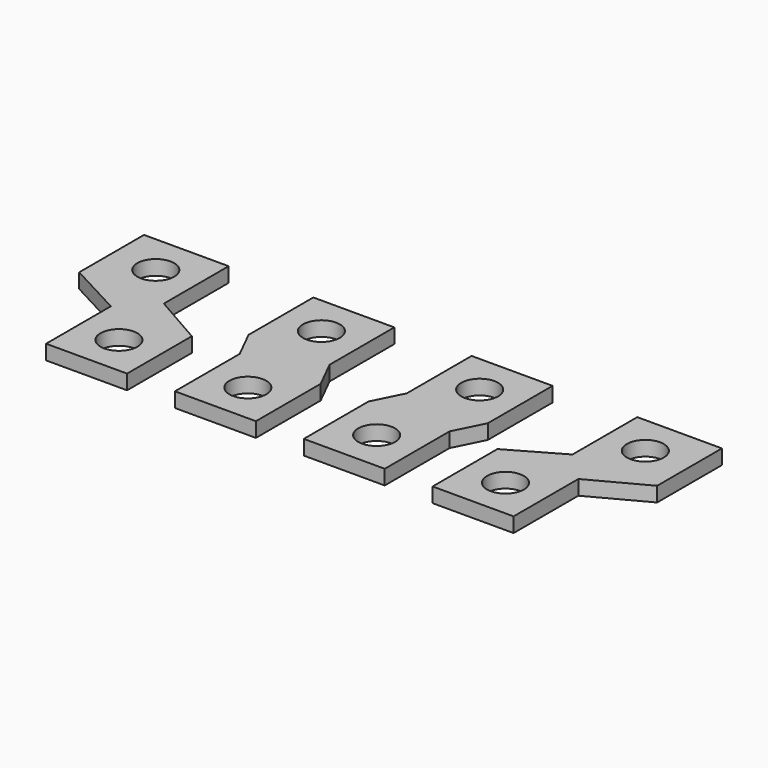
from build123d import *

# Parameters (mm, degrees)
F0_R     = 5
F1_DEPTH = 4


# Not quite as in the source:
# - a feature names something its author has since deleted; it is built from what else it names


with BuildPart() as f1:
    # F0 (on Top) → F1 (new body)
    with BuildSketch(Plane.XY):
        Polygon((-33.4400572926, 67.2019907534), (-56.4400572926, 67.2019907534), (-56.4400572926, 45.2019907534), (-41.4400572926, 37.2019907534), (-41.4400572926, 15.2019907534), (-19.4400572926, 15.2019907534), (-19.4400572926, 37.2019907534), (-33.4400572926, 45.2019907534), align=None)
        with Locations((-30.4400572926, 26.2019907534)):
            Circle(F0_R, mode=Mode.SUBTRACT)
        with Locations((-44.4400572926, 56.2019907534)):
            Circle(F0_R, mode=Mode.SUBTRACT)
    extrude(amount=F1_DEPTH)


with BuildPart() as f1b:
    # F0 (on Top) → F1, piece 2 (new body)
    with BuildSketch(Plane.XY):
        Polygon((11.5599427074, 67.2019907534), (-10.4400572926, 67.2019907534), (-10.4400572926, 45.2019907534), (-6.4400572926, 37.2019907534), (-6.4400572926, 15.2019907534), (15.5599427074, 15.2019907534), (15.5599427074, 25.1399558038), (15.5599427074, 37.2019907534), (11.5599427074, 45.2019907534), align=None)
        with Locations((4.5599427074, 26.2019907534)):
            Circle(F0_R, mode=Mode.SUBTRACT)
        with Locations((0.5599427074, 56.2019907534)):
            Circle(F0_R, mode=Mode.SUBTRACT)
    extrude(amount=F1_DEPTH)


with BuildPart() as f1c:
    # F0 (on Top) → F1, piece 3 (new body)
    with BuildSketch(Plane.XY):
        Polygon((28.5599427074, 15.2019907534), (50.5599427074, 15.2019907534), (50.5599427074, 37.2019907534), (54.5599427074, 45.2019907534), (54.5599427074, 67.2019907534), (32.5599427074, 67.2019907534), (32.5599427074, 45.2019907534), (28.5599427074, 37.2019907534), align=None)
        with Locations((39.5599427074, 26.2019907534)):
            Circle(F0_R, mode=Mode.SUBTRACT)
        with Locations((43.5599427074, 56.2019907534)):
            Circle(F0_R, mode=Mode.SUBTRACT)
    extrude(amount=F1_DEPTH)


with BuildPart() as f1d:
    # F0 (on Top) → F1, piece 4 (new body)
    with BuildSketch(Plane.XY):
        Polygon((77.5599427074, 67.2019907534), (77.5599427074, 45.2019907534), (63.5599427074, 37.2019907534), (63.5599427074, 15.2019907534), (85.5599427074, 15.2019907534), (85.5599427074, 37.2019907534), (100.5599427074, 45.2019907534), (100.5599427074, 67.2019907534), align=None)
        with Locations((74.5599427074, 26.2019907534)):
            Circle(F0_R, mode=Mode.SUBTRACT)
        with Locations((88.5599427074, 56.2019907534)):
            Circle(F0_R, mode=Mode.SUBTRACT)
    extrude(amount=F1_DEPTH)


solid = Compound([f1.part, f1b.part, f1c.part, f1d.part])
